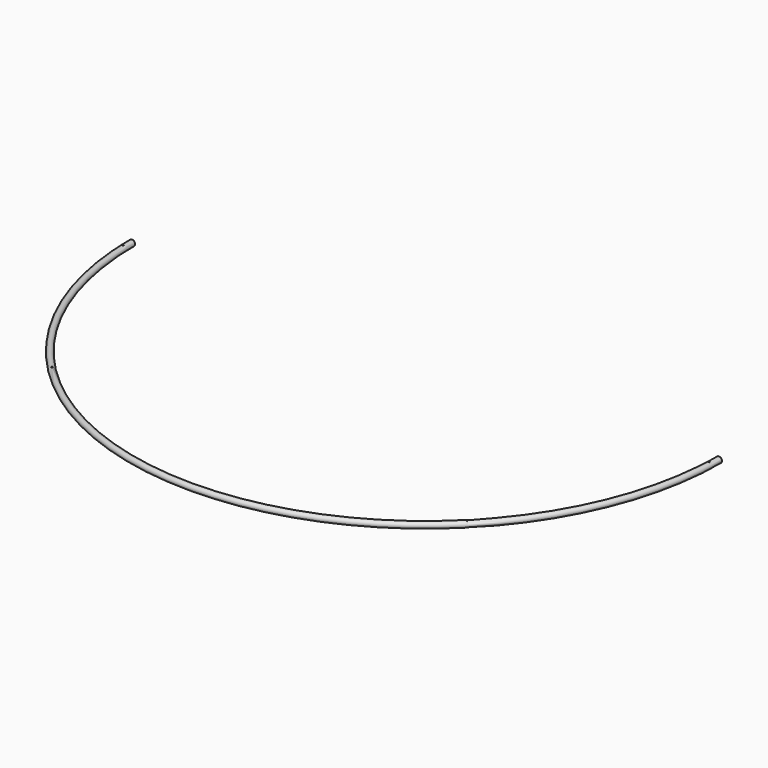
from build123d import *
from build123d import SkipClean  # not in build123d's __all__

# Parameters (mm, degrees)
F0_R          = 19.05
F0_R_2        = 15.85
F1_ANGLE      = 180
F2_R          = 5.25
F3_DEPTH      = 19.0510001
F3_DEPTH_BACK = 19.0510001
F4_R          = 5
F5_DEPTH      = 19.051000101
F5_DEPTH_BACK = 19.0510001007


with BuildPart() as f1:
    # F0 (on Front) → F1 (revolve)
    with BuildSketch(Plane.XZ):
        with Locations((-1850, 0)):
            Circle(F0_R)
        with Locations((-1850, 0)):
            Circle(F0_R_2, mode=Mode.SUBTRACT)
    revolve(axis=Axis((0, 0, 190.0846064091), (0, 0, 1)), revolution_arc=F1_ANGLE)

    # F2 (on Top) → F3 (cut, two sides)
    with BuildSketch(Plane.XY) as f3_sk:
        with Locations((-1848.4791045614, -75)):
            Circle(F2_R)
        with Locations((1848.4791045614, -75)):
            Circle(F2_R)
    with SkipClean():  # cleaning this boolean's faces spoils the solid; the shape is the same uncleaned
        extrude(amount=-F3_DEPTH, mode=Mode.SUBTRACT)
        extrude(f3_sk.sketch, amount=F3_DEPTH_BACK, mode=Mode.SUBTRACT)

    # F4 (on Top) → F5 (cut, two sides)
    with BuildSketch(Plane.XY) as f5_sk:
        with Locations((-1308.1475451951, -1308.1475451951)):
            Circle(F4_R)
        with Locations((1308.1475451951, -1308.1475451951)):
            Circle(F4_R)
    with SkipClean():  # cleaning this boolean's faces spoils the solid; the shape is the same uncleaned
        extrude(amount=F5_DEPTH, mode=Mode.SUBTRACT)
        extrude(f5_sk.sketch, amount=-F5_DEPTH_BACK, mode=Mode.SUBTRACT)


solid = f1.part
